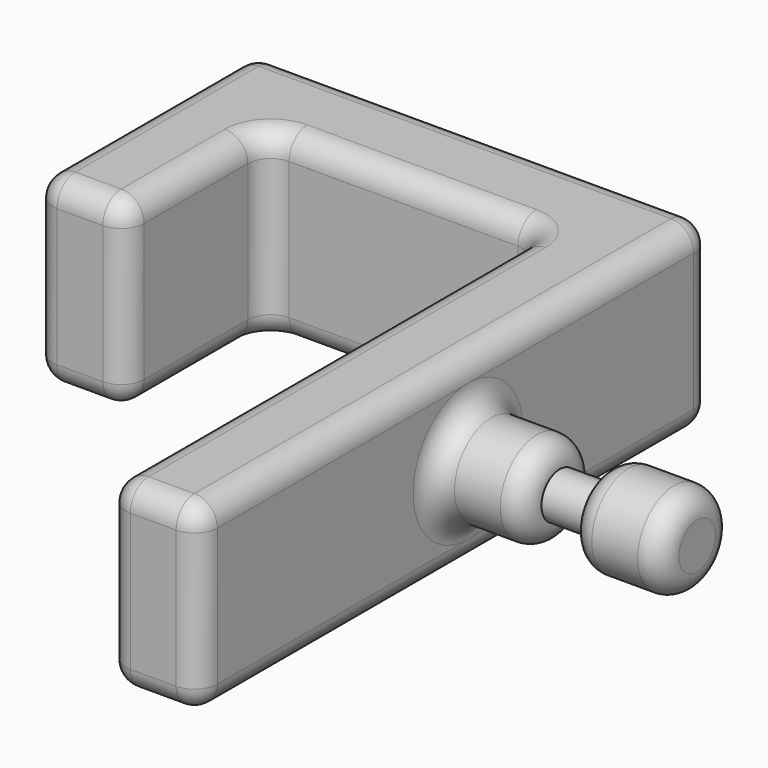
from build123d import *

# Parameters (mm, degrees)
F0_W          = 10
F0_H          = 10.8503269244
F0_W_2        = 30
F0_H_2        = 19.1496730756
F0_H_3        = 59.1496730756
F1_DEPTH      = 20
F2_R          = 5
F3_DEPTH      = 10
F5_R          = 2.5
F6_DEPTH      = 5
F7_R          = 5
F7_R_2        = 2.5
F8_DEPTH      = 10
F9_F1_R       = 2.5
F9_F2_R       = 2.5
F10_T3_DEPTH  = 5
F10_T5_DEPTH  = 5
F10_S9_W      = 2.5
F10_S9_H      = 2.5
F10_T10_DEPTH = 2.5
F10_S15_W     = 2.5
F10_S15_H     = 2.5
F10_T16_DEPTH = 2.5
F10_S21_W     = 2.5
F10_S21_H     = 2.5
F10_T22_DEPTH = 2.5
F10_S27_W     = 2.5
F10_S27_H     = 2.5
F10_T28_DEPTH = 2.5
F10_S33_W     = 2.5
F10_S33_H     = 2.5
F10_T34_DEPTH = 2.5
F10_S39_W     = 2.5
F10_S39_H     = 2.5
F10_T40_DEPTH = 2.5
F11_T1_DEPTH  = 5
F11_S5_W      = 2.5
F11_S5_H      = 2.5
F11_T6_DEPTH  = 2.5
F11_S11_W     = 2.5
F11_S11_H     = 2.5
F11_T12_DEPTH = 2.5


# Not quite as in the source:
# - a fillet or chamfer that OpenCascade refuses, or shapes differently, is made with other operations: its cross-section is extruded or revolved along the edge and cut away or added


with BuildPart() as f1:
    # F0 (on Top) → F1 (new body)
    with BuildSketch(Plane.XY):
        with Locations((-45, 27.8493528361)):
            Rectangle(F0_W, F0_H)
        with Locations((-25, 27.8493528361)):
            Rectangle(F0_W_2, F0_H)
        with Locations((-45, 12.8493528361)):
            Rectangle(F0_W, F0_H_2)
        with Locations((-5, 27.8493528361)):
            Rectangle(F0_W, F0_H)
        with Locations((-5, -7.1506471639)):
            Rectangle(F0_W, F0_H_3)
    extrude(amount=F1_DEPTH)

    # F2 (on face) → F3 (join)
    with BuildSketch(Plane.YZ):
        with Locations((0, 10)):
            Circle(F2_R)
    extrude(amount=F3_DEPTH)

    # F5 (on face) → F6 (join)
    with BuildSketch(Plane.YZ.offset(10)):
        with Locations((0, 10)):
            Circle(F5_R)
    extrude(amount=F6_DEPTH)

    # F7 (on face) → F8 (join)
    with BuildSketch(Plane.YZ.offset(15)):
        with Locations((0, 10)):
            Circle(F7_R)
        with Locations((0, 10)):
            Circle(F7_R_2, mode=Mode.SUBTRACT)
        with Locations((0, 10)):
            Circle(F7_R_2)
    extrude(amount=F8_DEPTH)

    # F9: fillet of radius 2.5 on 16 edges, made by hand

    # F9_f1
    f9_f1_edges = [f1.edges().sort_by_distance(p)[0] for p in [
        (-40, 22.4241893739, 10),
        (-10, 22.4241893739, 10),
    ]]
    fillet(f9_f1_edges, radius=F9_F1_R)

    # F9_f2
    f9_f2_edges = [f1.edges().sort_by_distance(p)[0] for p in [
        (0, 33.2745162983, 10),
        (-50, 33.2745162983, 10),
        (-50, 3.2745162983, 10),
        (-40, 3.2745162983, 10),
        (-10, -36.7254837017, 10),
        (0, -36.7254837017, 10),
        (0, -1.7254837017, 20),
        (-10, -8.4006471639, 20),
        (-25, 22.4241893739, 0),
        (-50, 18.2745162983, 20),
        (-50, 18.2745162983, 0),
        (-25, 33.2745162983, 0),
        (-25, 33.2745162983, 20),
        (0, -1.7254837017, 0),
        (-39.267766953, 21.6919563268, 0),
        (-10.732233047, 21.6919563268, 0),
        (-10.732233047, 21.6919563268, 20),
    ]]
    fillet(f9_f2_edges, radius=F9_F2_R)

    # F10: fillet of radius 2.5 on 7 edges, made by hand

    # F10_s1 → F10_t2 (revolve)
    with BuildSketch(Plane.XY.offset(10)):
        with BuildLine():
            ThreePointArc((0, 7.5), (0.732233047, 5.732233047), (2.5, 5))
            Line((2.5, 5), (0, 5))
            Line((0, 5), (0, 7.5))
        make_face()
    revolve(axis=Axis((0, 0, 10), (1, 0, 0)))

    # F10_s4 → F10_t3 (cut)
    with BuildSketch(Plane.YZ.offset(-47.5)):
        with BuildLine():
            ThreePointArc((5.7745162983, 0), (4.0067493453, 0.732233047), (3.2745162983, 2.5))
            Line((3.2745162983, 2.5), (3.2745162983, 0))
            Line((3.2745162983, 0), (5.7745162983, 0))
        make_face()
    extrude(amount=F10_T3_DEPTH, mode=Mode.SUBTRACT)

    # F10_s6 → F10_t5 (cut)
    with BuildSketch(Plane.YZ.offset(-7.5)):
        with BuildLine():
            ThreePointArc((-34.2254837017, 0), (-35.9932506547, 0.732233047), (-36.7254837017, 2.5))
            Line((-36.7254837017, 2.5), (-36.7254837017, 0))
            Line((-36.7254837017, 0), (-34.2254837017, 0))
        make_face()
        with BuildLine():
            ThreePointArc((-36.7254837017, 17.5), (-35.9932506547, 19.267766953), (-34.2254837017, 20))
            Line((-34.2254837017, 20), (-36.7254837017, 20))
            Line((-36.7254837017, 20), (-36.7254837017, 17.5))
        make_face()
    extrude(amount=F10_T5_DEPTH, mode=Mode.SUBTRACT)


with BuildPart() as f10_tool8:
    # F10_s9 → F10_t10 (new body)
    with BuildSketch(Plane.XZ.offset(34.2254837017)):
        with Locations((-8.75, 18.75)):
            Rectangle(F10_S9_W, F10_S9_H)
    extrude(amount=F10_T10_DEPTH)

    # F10_s11 → F10_t12 (revolve, cut)
    with BuildSketch(Plane(origin=(-7.5, -34.2254837017, 17.5), x_dir=(0.7071067812, 0, -0.7071067812), z_dir=(-0.7071067812, 0, -0.7071067812))):
        with BuildLine():
            ThreePointArc((0, -2.5), (2.5, 0), (0, 2.5))
            Line((0, 2.5), (0, -2.5))
        make_face()
    revolve(axis=Axis((-7.5, -34.2254837017, 17.5), (0, -1, 0)), mode=Mode.SUBTRACT)


with BuildPart() as f1_1:
    add(f1.part)

    # F10_t7: cut F10_tool8
    add(f10_tool8.part, mode=Mode.SUBTRACT)


with BuildPart() as f10_tool14:
    # F10_s15 → F10_t16 (new body)
    with BuildSketch(Plane.XZ.offset(34.2254837017)):
        with Locations((-1.25, 18.75)):
            Rectangle(F10_S15_W, F10_S15_H)
    extrude(amount=F10_T16_DEPTH)

    # F10_s17 → F10_t18 (revolve, cut)
    with BuildSketch(Plane(origin=(-2.5, -34.2254837017, 17.5), x_dir=(-0.7071067812, 0, -0.7071067812), z_dir=(-0.7071067812, 0, 0.7071067812))):
        with BuildLine():
            ThreePointArc((0, -2.5), (2.5, 0), (0, 2.5))
            Line((0, 2.5), (0, -2.5))
        make_face()
    revolve(axis=Axis((-2.5, -34.2254837017, 17.5), (0, -1, 0)), mode=Mode.SUBTRACT)


with BuildPart() as f1_2:
    add(f1_1.part)

    # F10_t13: cut F10_tool14
    add(f10_tool14.part, mode=Mode.SUBTRACT)


with BuildPart() as f10_tool20:
    # F10_s21 → F10_t22 (new body)
    with BuildSketch(Plane.XY.offset(2.5)):
        with Locations((-8.75, -35.4754837017)):
            Rectangle(F10_S21_W, F10_S21_H)
    extrude(amount=-F10_T22_DEPTH)

    # F10_s23 → F10_t24 (revolve, cut)
    with BuildSketch(Plane(origin=(-7.5, -34.2254837017, 2.5), x_dir=(0.7071067812, 0.7071067812, 0), z_dir=(-0.7071067812, 0.7071067812, 0))):
        with BuildLine():
            ThreePointArc((0, -2.5), (2.5, 0), (0, 2.5))
            Line((0, 2.5), (0, -2.5))
        make_face()
    revolve(axis=Axis((-7.5, -34.2254837017, 2.5), (0, 0, -1)), mode=Mode.SUBTRACT)


with BuildPart() as f1_3:
    add(f1_2.part)

    # F10_t19: cut F10_tool20
    add(f10_tool20.part, mode=Mode.SUBTRACT)


with BuildPart() as f10_tool26:
    # F10_s27 → F10_t28 (new body)
    with BuildSketch(Plane.XY.offset(2.5)):
        with Locations((-1.25, -35.4754837017)):
            Rectangle(F10_S27_W, F10_S27_H)
    extrude(amount=-F10_T28_DEPTH)

    # F10_s29 → F10_t30 (revolve, cut)
    with BuildSketch(Plane(origin=(-2.5, -34.2254837017, 2.5), x_dir=(-0.7071067812, 0.7071067812, 0), z_dir=(-0.7071067812, -0.7071067812, 0))):
        with BuildLine():
            ThreePointArc((0, -2.5), (2.5, 0), (0, 2.5))
            Line((0, 2.5), (0, -2.5))
        make_face()
    revolve(axis=Axis((-2.5, -34.2254837017, 2.5), (0, 0, -1)), mode=Mode.SUBTRACT)


with BuildPart() as f1_4:
    add(f1_3.part)

    # F10_t25: cut F10_tool26
    add(f10_tool26.part, mode=Mode.SUBTRACT)


with BuildPart() as f10_tool32:
    # F10_s33 → F10_t34 (new body)
    with BuildSketch(Plane.XY.offset(2.5)):
        with Locations((-48.75, 4.5245162983)):
            Rectangle(F10_S33_W, F10_S33_H)
    extrude(amount=-F10_T34_DEPTH)

    # F10_s35 → F10_t36 (revolve, cut)
    with BuildSketch(Plane(origin=(-47.5, 5.7745162983, 2.5), x_dir=(0.7071067812, 0.7071067812, 0), z_dir=(-0.7071067812, 0.7071067812, 0))):
        with BuildLine():
            ThreePointArc((0, -2.5), (2.5, 0), (0, 2.5))
            Line((0, 2.5), (0, -2.5))
        make_face()
    revolve(axis=Axis((-47.5, 5.7745162983, 2.5), (0, 0, -1)), mode=Mode.SUBTRACT)


with BuildPart() as f1_5:
    add(f1_4.part)

    # F10_t31: cut F10_tool32
    add(f10_tool32.part, mode=Mode.SUBTRACT)


with BuildPart() as f10_tool38:
    # F10_s39 → F10_t40 (new body)
    with BuildSketch(Plane.XY.offset(2.5)):
        with Locations((-41.25, 4.5245162983)):
            Rectangle(F10_S39_W, F10_S39_H)
    extrude(amount=-F10_T40_DEPTH)

    # F10_s41 → F10_t42 (revolve, cut)
    with BuildSketch(Plane(origin=(-42.5, 5.7745162983, 2.5), x_dir=(-0.7071067812, 0.7071067812, 0), z_dir=(-0.7071067812, -0.7071067812, 0))):
        with BuildLine():
            ThreePointArc((0, -2.5), (2.5, 0), (0, 2.5))
            Line((0, 2.5), (0, -2.5))
        make_face()
    revolve(axis=Axis((-42.5, 5.7745162983, 2.5), (0, 0, -1)), mode=Mode.SUBTRACT)


with BuildPart() as f1_6:
    add(f1_5.part)

    # F10_t37: cut F10_tool38
    add(f10_tool38.part, mode=Mode.SUBTRACT)

    # F10_s43 → F10_t44 (revolve, cut)
    with BuildSketch(Plane.XY.offset(10)):
        with BuildLine():
            ThreePointArc((22.5, 5), (24.267766953, 4.267766953), (25, 2.5))
            Line((25, 2.5), (25, 5))
            Line((25, 5), (22.5, 5))
        make_face()
    revolve(axis=Axis((25, 0, 10), (1, 0, 0)), mode=Mode.SUBTRACT)

    # F10_s45 → F10_t46 (revolve, cut)
    with BuildSketch(Plane.XY.offset(10)):
        with BuildLine():
            ThreePointArc((7.5, 5), (9.267766953, 4.267766953), (10, 2.5))
            Line((10, 2.5), (10, 5))
            Line((10, 5), (7.5, 5))
        make_face()
    revolve(axis=Axis((10, 0, 10), (1, 0, 0)), mode=Mode.SUBTRACT)

    # F10_s47 → F10_t48 (revolve, cut)
    with BuildSketch(Plane.XY.offset(10)):
        with BuildLine():
            ThreePointArc((15, 2.5), (15.732233047, 4.267766953), (17.5, 5))
            Line((17.5, 5), (15, 5))
            Line((15, 5), (15, 2.5))
        make_face()
    revolve(axis=Axis((15, 0, 10), (1, 0, 0)), mode=Mode.SUBTRACT)

    # F11: fillet of radius 2.5 on 1 edges, made by hand

    # F11_s2 → F11_t1 (cut)
    with BuildSketch(Plane.YZ.offset(-47.5)):
        with BuildLine():
            ThreePointArc((3.2745162983, 17.5), (4.0067493453, 19.267766953), (5.7745162983, 20))
            Line((5.7745162983, 20), (3.2745162983, 20))
            Line((3.2745162983, 20), (3.2745162983, 17.5))
        make_face()
    extrude(amount=F11_T1_DEPTH, mode=Mode.SUBTRACT)


with BuildPart() as f11_tool4:
    # F11_s5 → F11_t6 (new body)
    with BuildSketch(Plane.XZ.offset(-5.7745162983)):
        with Locations((-48.75, 18.75)):
            Rectangle(F11_S5_W, F11_S5_H)
    extrude(amount=F11_T6_DEPTH)

    # F11_s7 → F11_t8 (revolve, cut)
    with BuildSketch(Plane(origin=(-47.5, 5.7745162983, 17.5), x_dir=(0.7071067812, 0, -0.7071067812), z_dir=(-0.7071067812, 0, -0.7071067812))):
        with BuildLine():
            ThreePointArc((0, -2.5), (2.5, 0), (0, 2.5))
            Line((0, 2.5), (0, -2.5))
        make_face()
    revolve(axis=Axis((-47.5, 5.7745162983, 17.5), (0, -1, 0)), mode=Mode.SUBTRACT)


with BuildPart() as f1_7:
    add(f1_6.part)

    # F11_t3: cut F11_tool4
    add(f11_tool4.part, mode=Mode.SUBTRACT)


with BuildPart() as f11_tool10:
    # F11_s11 → F11_t12 (new body)
    with BuildSketch(Plane.XZ.offset(-5.7745162983)):
        with Locations((-41.25, 18.75)):
            Rectangle(F11_S11_W, F11_S11_H)
    extrude(amount=F11_T12_DEPTH)

    # F11_s13 → F11_t14 (revolve, cut)
    with BuildSketch(Plane(origin=(-42.5, 5.7745162983, 17.5), x_dir=(-0.7071067812, 0, -0.7071067812), z_dir=(-0.7071067812, 0, 0.7071067812))):
        with BuildLine():
            ThreePointArc((0, -2.5), (2.5, 0), (0, 2.5))
            Line((0, 2.5), (0, -2.5))
        make_face()
    revolve(axis=Axis((-42.5, 5.7745162983, 17.5), (0, -1, 0)), mode=Mode.SUBTRACT)


with BuildPart() as f1_8:
    add(f1_7.part)

    # F11_t9: cut F11_tool10
    add(f11_tool10.part, mode=Mode.SUBTRACT)


solid = f1_8.part
